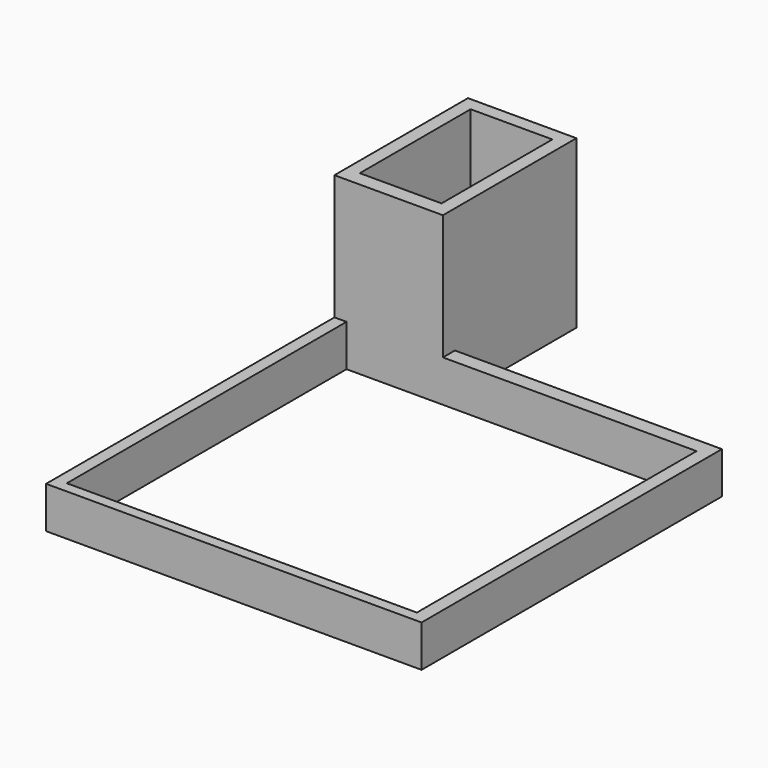
from build123d import *

# Parameters (mm, degrees)
F0_W     = 19.6
F0_H     = 33.2
F1_DEPTH = 40
F2_DEPTH = 10
F3_DEPTH = 2


# Not quite as in the source:
# - a feature names something its author has since deleted; it is built from what else it names


with BuildPart() as f1:
    # F0 (on Top) → F1 (new body)
    with BuildSketch(Plane.XY):
        Polygon((0, 0), (0, -3.6), (2.9, -3.6), (26, -3.6), (26, 0), (26, 36.4), (0, 36.4), align=None)
        with Locations((13, 16.6)):
            Rectangle(F0_W, F0_H, mode=Mode.SUBTRACT)
    extrude(amount=F1_DEPTH)

    # F0 (on Top) → F2 (join)
    with BuildSketch(Plane.XY):
        Polygon((86.8, -90), (90, -90), (90, -87.4), (90, 0), (26, 0), (26, -3.6), (86.8, -3.6), (86.8, -87.4), (2.9, -87.4), (2.9, -3.6), (0, -3.6), (0, -90), align=None)
    extrude(amount=F2_DEPTH)

    # F0 (on Top) → F3 (join)
    with BuildSketch(Plane.XY):
        with Locations((13, 16.6)):
            Rectangle(F0_W, F0_H)
    extrude(amount=F3_DEPTH)


solid = f1.part
